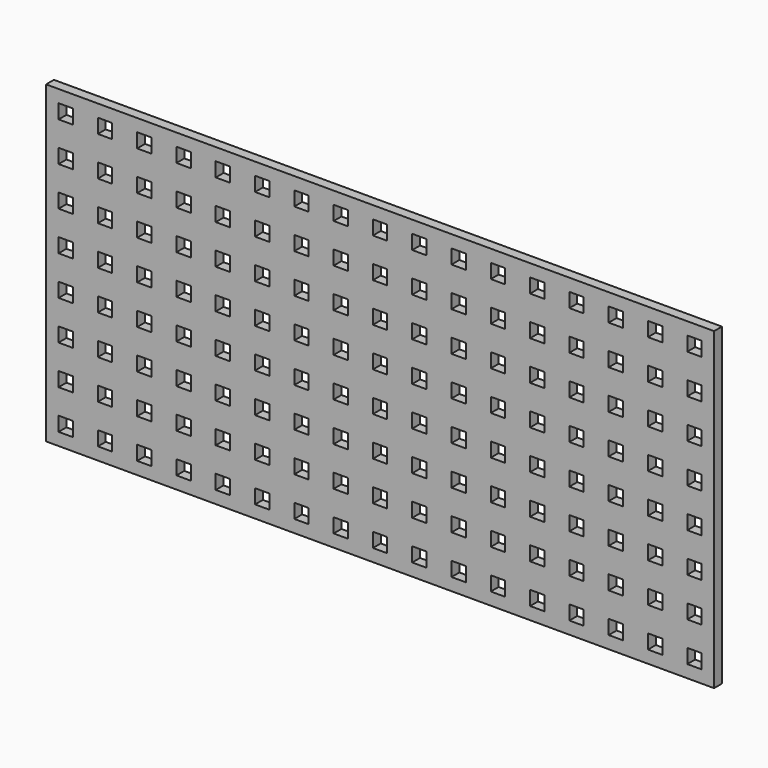
from build123d import *

# Parameters (mm, degrees)
F0_W     = 4.6228
F0_H     = 4.6228
F1_DEPTH = 3.175


# Not quite as in the source:
# - a length typed as a fraction of an inch, garbled in the dataset ("3 / 203.2 mm" for 3/8 in), is restored


with BuildPart() as f1:
    # F0 (on Front) → F1 (new body)
    with BuildSketch(Plane.XZ):
        Polygon((107.95, -50.8), (107.95, 50.8), (-107.95, 50.8), (-107.95, -44.45), (-107.95, -50.8), (-101.6, -50.8), align=None)
        with Locations((-101.6, -44.45)):
            Rectangle(F0_W, F0_H, mode=Mode.SUBTRACT)
        with Locations((-88.9, -44.45)):
            Rectangle(F0_W, F0_H, mode=Mode.SUBTRACT)
        with Locations((-76.2, -44.45)):
            Rectangle(F0_W, F0_H, mode=Mode.SUBTRACT)
        with Locations((-63.5, -44.45)):
            Rectangle(F0_W, F0_H, mode=Mode.SUBTRACT)
        with Locations((-101.6, -31.75)):
            Rectangle(F0_W, F0_H, mode=Mode.SUBTRACT)
        with Locations((-88.9, -31.75)):
            Rectangle(F0_W, F0_H, mode=Mode.SUBTRACT)
        with Locations((-76.2, -31.75)):
            Rectangle(F0_W, F0_H, mode=Mode.SUBTRACT)
        with Locations((-63.5, -31.75)):
            Rectangle(F0_W, F0_H, mode=Mode.SUBTRACT)
        with Locations((-50.8, -44.45)):
            Rectangle(F0_W, F0_H, mode=Mode.SUBTRACT)
        with Locations((-38.1, -44.45)):
            Rectangle(F0_W, F0_H, mode=Mode.SUBTRACT)
        with Locations((-25.4, -44.45)):
            Rectangle(F0_W, F0_H, mode=Mode.SUBTRACT)
        with Locations((-12.7, -44.45)):
            Rectangle(F0_W, F0_H, mode=Mode.SUBTRACT)
        with Locations((-50.8, -31.75)):
            Rectangle(F0_W, F0_H, mode=Mode.SUBTRACT)
        with Locations((-38.1, -31.75)):
            Rectangle(F0_W, F0_H, mode=Mode.SUBTRACT)
        with Locations((-25.4, -31.75)):
            Rectangle(F0_W, F0_H, mode=Mode.SUBTRACT)
        with Locations((-12.7, -31.75)):
            Rectangle(F0_W, F0_H, mode=Mode.SUBTRACT)
        with Locations((-101.6, -19.05)):
            Rectangle(F0_W, F0_H, mode=Mode.SUBTRACT)
        with Locations((-88.9, -19.05)):
            Rectangle(F0_W, F0_H, mode=Mode.SUBTRACT)
        with Locations((-76.2, -19.05)):
            Rectangle(F0_W, F0_H, mode=Mode.SUBTRACT)
        with Locations((-63.5, -19.05)):
            Rectangle(F0_W, F0_H, mode=Mode.SUBTRACT)
        with Locations((-101.6, -6.35)):
            Rectangle(F0_W, F0_H, mode=Mode.SUBTRACT)
        with Locations((-88.9, -6.35)):
            Rectangle(F0_W, F0_H, mode=Mode.SUBTRACT)
        with Locations((-76.2, -6.35)):
            Rectangle(F0_W, F0_H, mode=Mode.SUBTRACT)
        with Locations((-63.5, -6.35)):
            Rectangle(F0_W, F0_H, mode=Mode.SUBTRACT)
        with Locations((-50.8, -19.05)):
            Rectangle(F0_W, F0_H, mode=Mode.SUBTRACT)
        with Locations((-38.1, -19.05)):
            Rectangle(F0_W, F0_H, mode=Mode.SUBTRACT)
        with Locations((-25.4, -19.05)):
            Rectangle(F0_W, F0_H, mode=Mode.SUBTRACT)
        with Locations((-12.7, -19.05)):
            Rectangle(F0_W, F0_H, mode=Mode.SUBTRACT)
        with Locations((-50.8, -6.35)):
            Rectangle(F0_W, F0_H, mode=Mode.SUBTRACT)
        with Locations((-38.1, -6.35)):
            Rectangle(F0_W, F0_H, mode=Mode.SUBTRACT)
        with Locations((-25.4, -6.35)):
            Rectangle(F0_W, F0_H, mode=Mode.SUBTRACT)
        with Locations((-12.7, -6.35)):
            Rectangle(F0_W, F0_H, mode=Mode.SUBTRACT)
        with Locations((0, -44.45)):
            Rectangle(F0_W, F0_H, mode=Mode.SUBTRACT)
        with Locations((12.7, -44.45)):
            Rectangle(F0_W, F0_H, mode=Mode.SUBTRACT)
        with Locations((25.4, -44.45)):
            Rectangle(F0_W, F0_H, mode=Mode.SUBTRACT)
        with Locations((38.1, -44.45)):
            Rectangle(F0_W, F0_H, mode=Mode.SUBTRACT)
        with Locations((50.8, -44.45)):
            Rectangle(F0_W, F0_H, mode=Mode.SUBTRACT)
        with Locations((0, -31.75)):
            Rectangle(F0_W, F0_H, mode=Mode.SUBTRACT)
        with Locations((12.7, -31.75)):
            Rectangle(F0_W, F0_H, mode=Mode.SUBTRACT)
        with Locations((25.4, -31.75)):
            Rectangle(F0_W, F0_H, mode=Mode.SUBTRACT)
        with Locations((38.1, -31.75)):
            Rectangle(F0_W, F0_H, mode=Mode.SUBTRACT)
        with Locations((50.8, -31.75)):
            Rectangle(F0_W, F0_H, mode=Mode.SUBTRACT)
        with Locations((63.5, -44.45)):
            Rectangle(F0_W, F0_H, mode=Mode.SUBTRACT)
        with Locations((76.2, -44.45)):
            Rectangle(F0_W, F0_H, mode=Mode.SUBTRACT)
        with Locations((88.9, -44.45)):
            Rectangle(F0_W, F0_H, mode=Mode.SUBTRACT)
        with Locations((101.6, -44.45)):
            Rectangle(F0_W, F0_H, mode=Mode.SUBTRACT)
        with Locations((63.5, -31.75)):
            Rectangle(F0_W, F0_H, mode=Mode.SUBTRACT)
        with Locations((76.2, -31.75)):
            Rectangle(F0_W, F0_H, mode=Mode.SUBTRACT)
        with Locations((88.9, -31.75)):
            Rectangle(F0_W, F0_H, mode=Mode.SUBTRACT)
        with Locations((101.6, -31.75)):
            Rectangle(F0_W, F0_H, mode=Mode.SUBTRACT)
        with Locations((0, -19.05)):
            Rectangle(F0_W, F0_H, mode=Mode.SUBTRACT)
        with Locations((12.7, -19.05)):
            Rectangle(F0_W, F0_H, mode=Mode.SUBTRACT)
        with Locations((25.4, -19.05)):
            Rectangle(F0_W, F0_H, mode=Mode.SUBTRACT)
        with Locations((38.1, -19.05)):
            Rectangle(F0_W, F0_H, mode=Mode.SUBTRACT)
        with Locations((50.8, -19.05)):
            Rectangle(F0_W, F0_H, mode=Mode.SUBTRACT)
        with Locations((0, -6.35)):
            Rectangle(F0_W, F0_H, mode=Mode.SUBTRACT)
        with Locations((12.7, -6.35)):
            Rectangle(F0_W, F0_H, mode=Mode.SUBTRACT)
        with Locations((25.4, -6.35)):
            Rectangle(F0_W, F0_H, mode=Mode.SUBTRACT)
        with Locations((38.1, -6.35)):
            Rectangle(F0_W, F0_H, mode=Mode.SUBTRACT)
        with Locations((50.8, -6.35)):
            Rectangle(F0_W, F0_H, mode=Mode.SUBTRACT)
        with Locations((63.5, -19.05)):
            Rectangle(F0_W, F0_H, mode=Mode.SUBTRACT)
        with Locations((76.2, -19.05)):
            Rectangle(F0_W, F0_H, mode=Mode.SUBTRACT)
        with Locations((88.9, -19.05)):
            Rectangle(F0_W, F0_H, mode=Mode.SUBTRACT)
        with Locations((101.6, -19.05)):
            Rectangle(F0_W, F0_H, mode=Mode.SUBTRACT)
        with Locations((63.5, -6.35)):
            Rectangle(F0_W, F0_H, mode=Mode.SUBTRACT)
        with Locations((76.2, -6.35)):
            Rectangle(F0_W, F0_H, mode=Mode.SUBTRACT)
        with Locations((88.9, -6.35)):
            Rectangle(F0_W, F0_H, mode=Mode.SUBTRACT)
        with Locations((101.6, -6.35)):
            Rectangle(F0_W, F0_H, mode=Mode.SUBTRACT)
        with Locations((-101.6, 6.35)):
            Rectangle(F0_W, F0_H, mode=Mode.SUBTRACT)
        with Locations((-88.9, 6.35)):
            Rectangle(F0_W, F0_H, mode=Mode.SUBTRACT)
        with Locations((-76.2, 6.35)):
            Rectangle(F0_W, F0_H, mode=Mode.SUBTRACT)
        with Locations((-63.5, 6.35)):
            Rectangle(F0_W, F0_H, mode=Mode.SUBTRACT)
        with Locations((-101.6, 19.05)):
            Rectangle(F0_W, F0_H, mode=Mode.SUBTRACT)
        with Locations((-88.9, 19.05)):
            Rectangle(F0_W, F0_H, mode=Mode.SUBTRACT)
        with Locations((-76.2, 19.05)):
            Rectangle(F0_W, F0_H, mode=Mode.SUBTRACT)
        with Locations((-63.5, 19.05)):
            Rectangle(F0_W, F0_H, mode=Mode.SUBTRACT)
        with Locations((-50.8, 6.35)):
            Rectangle(F0_W, F0_H, mode=Mode.SUBTRACT)
        with Locations((-38.1, 6.35)):
            Rectangle(F0_W, F0_H, mode=Mode.SUBTRACT)
        with Locations((-25.4, 6.35)):
            Rectangle(F0_W, F0_H, mode=Mode.SUBTRACT)
        with Locations((-12.7, 6.35)):
            Rectangle(F0_W, F0_H, mode=Mode.SUBTRACT)
        with Locations((-50.8, 19.05)):
            Rectangle(F0_W, F0_H, mode=Mode.SUBTRACT)
        with Locations((-38.1, 19.05)):
            Rectangle(F0_W, F0_H, mode=Mode.SUBTRACT)
        with Locations((-25.4, 19.05)):
            Rectangle(F0_W, F0_H, mode=Mode.SUBTRACT)
        with Locations((-12.7, 19.05)):
            Rectangle(F0_W, F0_H, mode=Mode.SUBTRACT)
        with Locations((-101.6, 31.75)):
            Rectangle(F0_W, F0_H, mode=Mode.SUBTRACT)
        with Locations((-88.9, 31.75)):
            Rectangle(F0_W, F0_H, mode=Mode.SUBTRACT)
        with Locations((-76.2, 31.75)):
            Rectangle(F0_W, F0_H, mode=Mode.SUBTRACT)
        with Locations((-63.5, 31.75)):
            Rectangle(F0_W, F0_H, mode=Mode.SUBTRACT)
        with Locations((-101.6, 44.45)):
            Rectangle(F0_W, F0_H, mode=Mode.SUBTRACT)
        with Locations((-88.9, 44.45)):
            Rectangle(F0_W, F0_H, mode=Mode.SUBTRACT)
        with Locations((-76.2, 44.45)):
            Rectangle(F0_W, F0_H, mode=Mode.SUBTRACT)
        with Locations((-63.5, 44.45)):
            Rectangle(F0_W, F0_H, mode=Mode.SUBTRACT)
        with Locations((-50.8, 31.75)):
            Rectangle(F0_W, F0_H, mode=Mode.SUBTRACT)
        with Locations((-38.1, 31.75)):
            Rectangle(F0_W, F0_H, mode=Mode.SUBTRACT)
        with Locations((-25.4, 31.75)):
            Rectangle(F0_W, F0_H, mode=Mode.SUBTRACT)
        with Locations((-12.7, 31.75)):
            Rectangle(F0_W, F0_H, mode=Mode.SUBTRACT)
        with Locations((-50.8, 44.45)):
            Rectangle(F0_W, F0_H, mode=Mode.SUBTRACT)
        with Locations((-38.1, 44.45)):
            Rectangle(F0_W, F0_H, mode=Mode.SUBTRACT)
        with Locations((-25.4, 44.45)):
            Rectangle(F0_W, F0_H, mode=Mode.SUBTRACT)
        with Locations((-12.7, 44.45)):
            Rectangle(F0_W, F0_H, mode=Mode.SUBTRACT)
        with Locations((0, 6.35)):
            Rectangle(F0_W, F0_H, mode=Mode.SUBTRACT)
        with Locations((12.7, 6.35)):
            Rectangle(F0_W, F0_H, mode=Mode.SUBTRACT)
        with Locations((25.4, 6.35)):
            Rectangle(F0_W, F0_H, mode=Mode.SUBTRACT)
        with Locations((38.1, 6.35)):
            Rectangle(F0_W, F0_H, mode=Mode.SUBTRACT)
        with Locations((50.8, 6.35)):
            Rectangle(F0_W, F0_H, mode=Mode.SUBTRACT)
        with Locations((0, 19.05)):
            Rectangle(F0_W, F0_H, mode=Mode.SUBTRACT)
        with Locations((12.7, 19.05)):
            Rectangle(F0_W, F0_H, mode=Mode.SUBTRACT)
        with Locations((25.4, 19.05)):
            Rectangle(F0_W, F0_H, mode=Mode.SUBTRACT)
        with Locations((38.1, 19.05)):
            Rectangle(F0_W, F0_H, mode=Mode.SUBTRACT)
        with Locations((50.8, 19.05)):
            Rectangle(F0_W, F0_H, mode=Mode.SUBTRACT)
        with Locations((63.5, 6.35)):
            Rectangle(F0_W, F0_H, mode=Mode.SUBTRACT)
        with Locations((76.2, 6.35)):
            Rectangle(F0_W, F0_H, mode=Mode.SUBTRACT)
        with Locations((88.9, 6.35)):
            Rectangle(F0_W, F0_H, mode=Mode.SUBTRACT)
        with Locations((101.6, 6.35)):
            Rectangle(F0_W, F0_H, mode=Mode.SUBTRACT)
        with Locations((63.5, 19.05)):
            Rectangle(F0_W, F0_H, mode=Mode.SUBTRACT)
        with Locations((76.2, 19.05)):
            Rectangle(F0_W, F0_H, mode=Mode.SUBTRACT)
        with Locations((88.9, 19.05)):
            Rectangle(F0_W, F0_H, mode=Mode.SUBTRACT)
        with Locations((101.6, 19.05)):
            Rectangle(F0_W, F0_H, mode=Mode.SUBTRACT)
        with Locations((0, 31.75)):
            Rectangle(F0_W, F0_H, mode=Mode.SUBTRACT)
        with Locations((12.7, 31.75)):
            Rectangle(F0_W, F0_H, mode=Mode.SUBTRACT)
        with Locations((25.4, 31.75)):
            Rectangle(F0_W, F0_H, mode=Mode.SUBTRACT)
        with Locations((38.1, 31.75)):
            Rectangle(F0_W, F0_H, mode=Mode.SUBTRACT)
        with Locations((50.8, 31.75)):
            Rectangle(F0_W, F0_H, mode=Mode.SUBTRACT)
        with Locations((0, 44.45)):
            Rectangle(F0_W, F0_H, mode=Mode.SUBTRACT)
        with Locations((12.7, 44.45)):
            Rectangle(F0_W, F0_H, mode=Mode.SUBTRACT)
        with Locations((25.4, 44.45)):
            Rectangle(F0_W, F0_H, mode=Mode.SUBTRACT)
        with Locations((38.1, 44.45)):
            Rectangle(F0_W, F0_H, mode=Mode.SUBTRACT)
        with Locations((50.8, 44.45)):
            Rectangle(F0_W, F0_H, mode=Mode.SUBTRACT)
        with Locations((63.5, 31.75)):
            Rectangle(F0_W, F0_H, mode=Mode.SUBTRACT)
        with Locations((76.2, 31.75)):
            Rectangle(F0_W, F0_H, mode=Mode.SUBTRACT)
        with Locations((88.9, 31.75)):
            Rectangle(F0_W, F0_H, mode=Mode.SUBTRACT)
        with Locations((101.6, 31.75)):
            Rectangle(F0_W, F0_H, mode=Mode.SUBTRACT)
        with Locations((63.5, 44.45)):
            Rectangle(F0_W, F0_H, mode=Mode.SUBTRACT)
        with Locations((76.2, 44.45)):
            Rectangle(F0_W, F0_H, mode=Mode.SUBTRACT)
        with Locations((88.9, 44.45)):
            Rectangle(F0_W, F0_H, mode=Mode.SUBTRACT)
        with Locations((101.6, 44.45)):
            Rectangle(F0_W, F0_H, mode=Mode.SUBTRACT)
    extrude(amount=F1_DEPTH)


solid = f1.part
